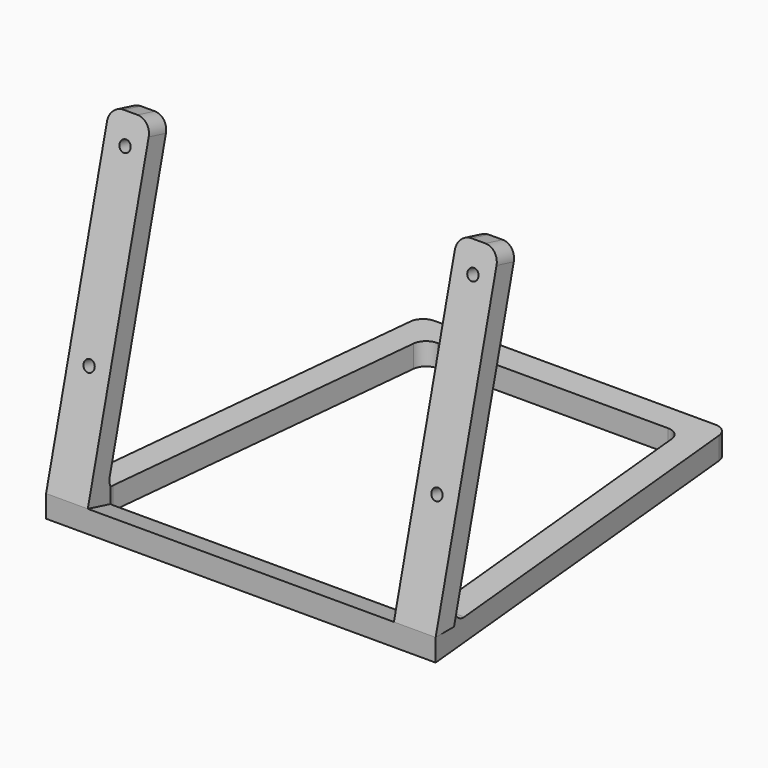
from build123d import *

# Parameters (mm, degrees)
F1_DEPTH      = 8
F3_DEPTH      = 70
F3_DEPTH_BACK = 70
F4_W          = 110
F4_H          = 115
F4_R          = 2
F5_DEPTH      = 10.5877977107
F6_R          = 5
F7_R          = 5


with BuildPart() as f1:
    # F0 (on Top) → F1 (new body)
    with BuildSketch(Plane.XY):
        with BuildLine():
            Line((-55.4502481405, 98.6044170713), (-70, -46.8931015238))
            Line((-70, -46.8931015238), (70, -46.8931015238))
            Line((70, -46.8931015238), (55.4502481405, 98.6044170713))
            ThreePointArc((55.4502481405, 98.6044170713), (53.8300887932, 101.8141611439), (50.4750621894, 103.1068984762))
            Line((50.4750621894, 103.1068984762), (-50.4750621894, 103.1068984762))
            ThreePointArc((-50.4750621894, 103.1068984762), (-53.8300887932, 101.8141611439), (-55.4502481405, 98.6044170713))
        make_face()
        with BuildLine():
            Line((-41.4251865683, 93.1068984762), (41.4251865683, 93.1068984762))
            ThreePointArc((41.4251865683, 93.1068984762), (44.7802131721, 91.8141611439), (46.4003725194, 88.6044170713))
            Line((46.4003725194, 88.6044170713), (58.4003725194, -31.3955829287))
            ThreePointArc((58.4003725194, -31.3955829287), (57.1324492361, -35.2481281276), (53.4251865683, -36.8931015238))
            Line((53.4251865683, -36.8931015238), (-53.4251865683, -36.8931015238))
            ThreePointArc((-53.4251865683, -36.8931015238), (-57.1324492361, -35.2481281276), (-58.4003725194, -31.3955829287))
            Line((-58.4003725194, -31.3955829287), (-46.4003725194, 88.6044170713))
            ThreePointArc((-46.4003725194, 88.6044170713), (-44.7802131721, 91.8141611439), (-41.4251865683, 93.1068984762))
        make_face(mode=Mode.SUBTRACT)
    extrude(amount=F1_DEPTH)

    # F2 (on Right) → F3 (join, two sides)
    with BuildSketch(Plane.YZ) as f3_sk:
        Polygon((-18.3058557984, 119.3901673481), (-46.8931015238, 8), (-38.633844698, 8), (-35.4294686048, 20.4858474544), (-10.5569745916, 117.4014893846), align=None)
    extrude(amount=F3_DEPTH)
    extrude(f3_sk.sketch, amount=-F3_DEPTH_BACK)

    # F4 (on face) → F5 (cut, through all)
    with BuildSketch(Plane(origin=(0, -45.9216252544, 11.7853560733), x_dir=(1, 0, 0), z_dir=(0, -0.9686101509, 0.2485847454))):
        with Locations((0, 53.5919715017)):
            Rectangle(F4_W, F4_H)
        with Locations((-62.5, 101.0919715017)):
            Circle(F4_R)
        with Locations((-62.5, 36.0919715017)):
            Circle(F4_R)
        with Locations((62.5, 36.0919715017)):
            Circle(F4_R)
        with Locations((62.5, 101.0919715017)):
            Circle(F4_R)
    extrude(amount=-F5_DEPTH, mode=Mode.SUBTRACT)

    # F6
    f6_edges = [f1.edges().sort_by_distance(p)[0] for p in [
        (-70, -14.431415, 118.395828),
        (-55, -14.431415, 118.395828),
        (55, -14.431415, 118.395828),
        (70, -14.431415, 118.395828),
    ]]
    fillet(f6_edges, radius=F6_R)

    # F7
    f7_edges = [f1.edges().sort_by_distance(p)[0] for p in [
        (-62.087037, -38.633845, 8),
        (62.087037, -38.633845, 8),
    ]]
    fillet(f7_edges, radius=F7_R)


solid = f1.part
